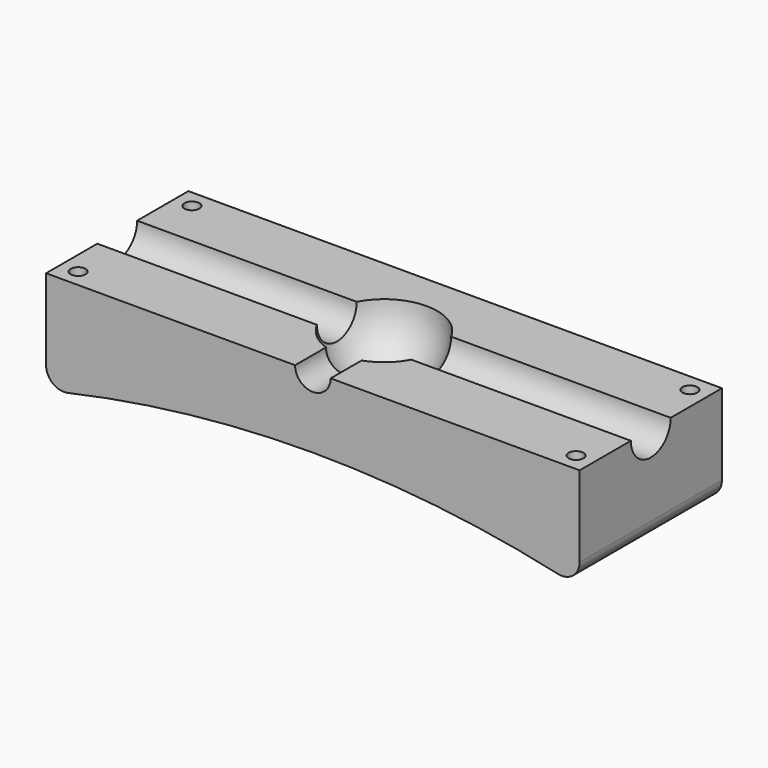
from build123d import *

# Parameters (mm, degrees)
F1_DEPTH = 25
F5_D     = 4.2
F5_DEPTH = 20
F5_TIP   = 1.2618073
F6_R     = 5


with BuildPart() as f1:
    # F0 (on Front) → F1 (new body, symmetric)
    with BuildSketch(Plane.XZ):
        with BuildLine():
            ThreePointArc((0, 315), (37.7725508345, 312.7270925319), (75, 305.9411708156))
            Line((75, 305.9411708156), (75, 335))
            Line((75, 335), (0, 335))
            Line((0, 335), (0, 315))
        make_face()
        with BuildLine():
            ThreePointArc((-75, 305.9411708156), (-37.7725508345, 312.7270925319), (0, 315))
            Line((0, 315), (0, 335))
            Line((0, 335), (-75, 335))
            Line((-75, 335), (-75, 305.9411708156))
        make_face()
    extrude(amount=F1_DEPTH, both=True)

    # F2 (on face) → F3 (revolve, cut)
    with BuildSketch(Plane.XY.offset(335)):
        with BuildLine():
            Line((-13.2664991614, 7), (-75, 7))
            Line((-75, 7), (-75, 0))
            Line((-75, 0), (-15, 0))
            ThreePointArc((-15, 0), (-14.5601766373, 3.6057254872), (-13.2664991614, 7))
        make_face()
        with BuildLine():
            ThreePointArc((13.2664991614, 7), (0, 15), (-13.2664991614, 7))
            ThreePointArc((-13.2664991614, 7), (-14.5601766373, 3.6057254872), (-15, 0))
            Line((-15, 0), (-13.2664991614, 0))
            Line((-13.2664991614, 0), (13.2664991614, 0))
            Line((13.2664991614, 0), (15, 0))
            ThreePointArc((15, 0), (14.5601766373, 3.6057254872), (13.2664991614, 7))
        make_face()
        with BuildLine():
            Line((75, 7), (13.2664991614, 7))
            ThreePointArc((13.2664991614, 7), (14.5601766373, 3.6057254872), (15, 0))
            Line((15, 0), (75, 0))
            Line((75, 0), (75, 7))
        make_face()
    revolve(axis=Axis((-44.1332495807, 0, 335), (1, 0, 0)), mode=Mode.SUBTRACT)

    # F5
    with Locations(Plane.XY.offset(335)):
        with Locations((-70, 20), (-70, -20), (70, 20), (70, -20)):
            Hole(F5_D / 2, depth=F5_DEPTH)
            with Locations((0, 0, -(F5_DEPTH + F5_TIP / 2))):  # 118° drill point
                Cone(0, F5_D / 2, F5_TIP, mode=Mode.SUBTRACT)

    # F6
    f6_edges = [f1.edges().sort_by_distance(p)[0] for p in [
        (-75, 0, 305.941171),
        (75, 0, 305.941171),
    ]]
    fillet(f6_edges, radius=F6_R)

    # F7 (on face) → F8 (revolve, cut)
    with BuildSketch(Plane.XY.offset(335)):
        with BuildLine():
            Line((0, 0), (-5, 0))
            Line((-5, 0), (-5, -14.1421356237))
            ThreePointArc((-5, -14.1421356237), (-2.5365296809, -14.7839783948), (0, -15))
            Line((0, -15), (0, 0))
        make_face()
        with BuildLine():
            ThreePointArc((0, -15), (-2.5365296809, -14.7839783948), (-5, -14.1421356237))
            Line((-5, -14.1421356237), (-5, -25))
            Line((-5, -25), (0, -25))
            Line((0, -25), (0, -15))
        make_face()
    revolve(axis=Axis((0, -12.5, 335), (0, -1, 0)), mode=Mode.SUBTRACT)


solid = f1.part
